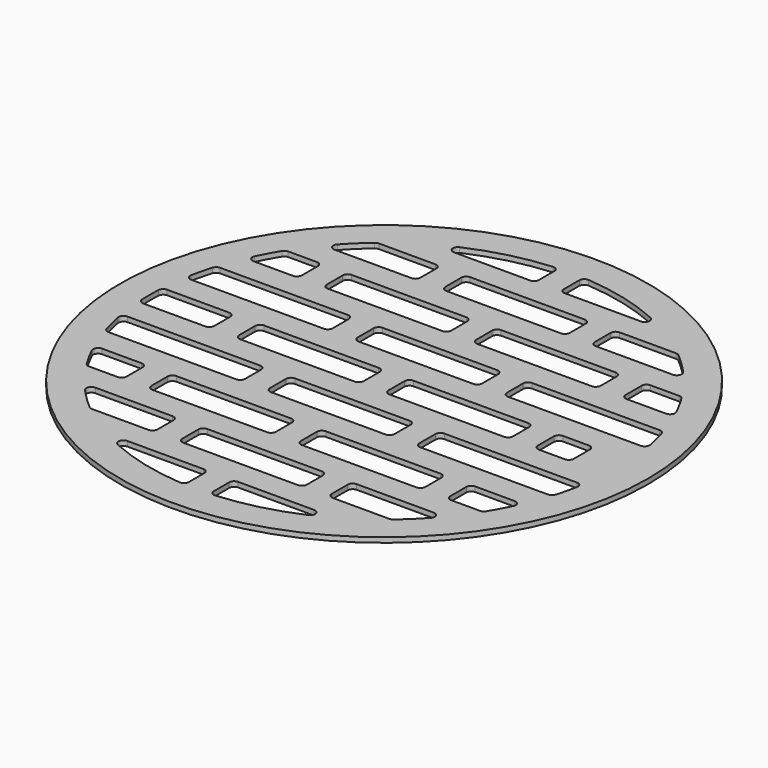
from build123d import *

# Parameters (mm, degrees)
F0_R     = 53
F0_W     = 25
F0_H     = 6
F0_W_2   = 7.2020787991
F1_DEPTH = 1
F2_R     = 1


with BuildPart() as f1:
    # F0 (on Top) → F1 (new body)
    with BuildSketch(Plane.XY):
        Circle(F0_R)
        with BuildLine():
            Line((-17.5, -30), (-17.5, -36))
            Line((-17.5, -36), (-30.2158898595, -36))
            ThreePointArc((-30.2158898595, -36), (-33.3332721818, -33.1344679398), (-36.1801050303, -30))
            Line((-36.1801050303, -30), (-17.5, -30))
        make_face(mode=Mode.SUBTRACT)
        with BuildLine():
            Line((-2.5, -41), (-2.5, -46.9334635415))
            ThreePointArc((-2.5, -46.9334635415), (-13.0800156969, -45.1432518697), (-22.9782505862, -41))
            Line((-22.9782505862, -41), (-2.5, -41))
        make_face(mode=Mode.SUBTRACT)
        with BuildLine():
            Line((-32.5, -25), (-39.7994974843, -25))
            ThreePointArc((-39.7994974843, -25), (-41.5025032039, -22.0577022332), (-42.9883705204, -19))
            Line((-42.9883705204, -19), (-32.5, -19))
            Line((-32.5, -19), (-32.5, -25))
        make_face(mode=Mode.SUBTRACT)
        with BuildLine():
            Line((-17.5, -14), (-44.8664685483, -14))
            ThreePointArc((-44.8664685483, -14), (-45.6889052007, -11.0237898005), (-46.3141447076, -8))
            Line((-46.3141447076, -8), (-17.5, -8))
            Line((-17.5, -8), (-17.5, -14))
        make_face(mode=Mode.SUBTRACT)
        with Locations((-15, -22)):
            Rectangle(F0_W, F0_H, mode=Mode.SUBTRACT)
        with BuildLine():
            ThreePointArc((22.9782505862, -41), (13.0800156969, -45.1432518697), (2.5, -46.9334635415))
            Line((2.5, -46.9334635415), (2.5, -41))
            Line((2.5, -41), (22.9782505862, -41))
        make_face(mode=Mode.SUBTRACT)
        with Locations((0, -33)):
            Rectangle(F0_W, F0_H, mode=Mode.SUBTRACT)
        with BuildLine():
            Line((30.2158898595, -36), (17.5, -36))
            Line((17.5, -36), (17.5, -30))
            Line((17.5, -30), (36.1801050303, -30))
            ThreePointArc((36.1801050303, -30), (33.3332721818, -33.1344679398), (30.2158898595, -36))
        make_face(mode=Mode.SUBTRACT)
        with Locations((15, -22)):
            Rectangle(F0_W, F0_H, mode=Mode.SUBTRACT)
        with Locations((0, -11)):
            Rectangle(F0_W, F0_H, mode=Mode.SUBTRACT)
        with BuildLine():
            Line((32.5, -19), (42.9883705204, -19))
            ThreePointArc((42.9883705204, -19), (41.5025032039, -22.0577022332), (39.7994974843, -25))
            Line((39.7994974843, -25), (32.5, -25))
            Line((32.5, -25), (32.5, -19))
        make_face(mode=Mode.SUBTRACT)
        with BuildLine():
            Line((17.5, -8), (46.3141447076, -8))
            ThreePointArc((46.3141447076, -8), (45.6889052007, -11.0237898005), (44.8664685483, -14))
            Line((44.8664685483, -14), (17.5, -14))
            Line((17.5, -14), (17.5, -8))
        make_face(mode=Mode.SUBTRACT)
        with BuildLine():
            Line((-32.5, -3), (-46.9041575982, -3))
            ThreePointArc((-46.9041575982, -3), (-47, 0), (-46.9041575982, 3))
            Line((-46.9041575982, 3), (-32.5, 3))
            Line((-32.5, 3), (-32.5, -3))
        make_face(mode=Mode.SUBTRACT)
        with BuildLine():
            Line((-17.5, 8), (-46.3141447076, 8))
            ThreePointArc((-46.3141447076, 8), (-45.6889052007, 11.0237898005), (-44.8664685483, 14))
            Line((-44.8664685483, 14), (-17.5, 14))
            Line((-17.5, 14), (-17.5, 8))
        make_face(mode=Mode.SUBTRACT)
        with BuildLine():
            Line((-32.5, 19), (-42.9883705204, 19))
            ThreePointArc((-42.9883705204, 19), (-41.5025032039, 22.0577022332), (-39.7994974843, 25))
            Line((-39.7994974843, 25), (-32.5, 25))
            Line((-32.5, 25), (-32.5, 19))
        make_face(mode=Mode.SUBTRACT)
        with Locations((-15, 0)):
            Rectangle(F0_W, F0_H, mode=Mode.SUBTRACT)
        with Locations((-15, 22)):
            Rectangle(F0_W, F0_H, mode=Mode.SUBTRACT)
        with BuildLine():
            Line((-17.5, 30), (-36.1801050303, 30))
            ThreePointArc((-36.1801050303, 30), (-33.3332721818, 33.1344679398), (-30.2158898595, 36))
            Line((-30.2158898595, 36), (-17.5, 36))
            Line((-17.5, 36), (-17.5, 30))
        make_face(mode=Mode.SUBTRACT)
        with BuildLine():
            ThreePointArc((-22.9782505862, 41), (-13.0800156969, 45.1432518697), (-2.5, 46.9334635415))
            Line((-2.5, 46.9334635415), (-2.5, 41))
            Line((-2.5, 41), (-22.9782505862, 41))
        make_face(mode=Mode.SUBTRACT)
        with Locations((0, 11)):
            Rectangle(F0_W, F0_H, mode=Mode.SUBTRACT)
        with Locations((15, 0)):
            Rectangle(F0_W, F0_H, mode=Mode.SUBTRACT)
        with Locations((15, 22)):
            Rectangle(F0_W, F0_H, mode=Mode.SUBTRACT)
        with Locations((36.1010393996, 0)):
            Rectangle(F0_W_2, F0_H, mode=Mode.SUBTRACT)
        with BuildLine():
            ThreePointArc((44.8664685483, 14), (45.6889052007, 11.0237898005), (46.3141447076, 8))
            Line((46.3141447076, 8), (17.5, 8))
            Line((17.5, 8), (17.5, 14))
            Line((17.5, 14), (44.8664685483, 14))
        make_face(mode=Mode.SUBTRACT)
        with BuildLine():
            ThreePointArc((39.7994974843, 25), (41.5025032039, 22.0577022332), (42.9883705204, 19))
            Line((42.9883705204, 19), (32.5, 19))
            Line((32.5, 19), (32.5, 25))
            Line((32.5, 25), (39.7994974843, 25))
        make_face(mode=Mode.SUBTRACT)
        with Locations((0, 33)):
            Rectangle(F0_W, F0_H, mode=Mode.SUBTRACT)
        with BuildLine():
            ThreePointArc((2.5, 46.9334635415), (13.0800156969, 45.1432518697), (22.9782505862, 41))
            Line((22.9782505862, 41), (2.5, 41))
            Line((2.5, 41), (2.5, 46.9334635415))
        make_face(mode=Mode.SUBTRACT)
        with BuildLine():
            ThreePointArc((30.2158898595, 36), (33.3332721818, 33.1344679398), (36.1801050303, 30))
            Line((36.1801050303, 30), (17.5, 30))
            Line((17.5, 30), (17.5, 36))
            Line((17.5, 36), (30.2158898595, 36))
        make_face(mode=Mode.SUBTRACT)
    extrude(amount=F1_DEPTH)

    # F2
    f2_edges = [f1.edges().sort_by_distance(p)[0] for p in [
        (22.978251, 41, 0.5),
        (-22.978251, 41, 0.5),
        (36.180105, 30, 0.5),
        (42.988371, 19, 0.5),
        (46.314145, 8, 0.5),
        (46.314145, -8, 0.5),
        (44.866469, -14, 0.5),
        (39.799497, -25, 0.5),
        (30.21589, -36, 0.5),
        (22.978251, -41, 0.5),
        (36.180105, -30, 0.5),
        (42.988371, -19, 0.5),
        (44.866469, 14, 0.5),
        (39.799497, 25, 0.5),
        (30.21589, 36, 0.5),
        (-2.5, 46.933464, 0.5),
        (-2.5, 41, 0.5),
        (2.5, 46.933464, 0.5),
        (2.5, 41, 0.5),
        (-36.180105, 30, 0.5),
        (-30.21589, 36, 0.5),
        (-17.5, 36, 0.5),
        (-17.5, 30, 0.5),
        (-2.5, 19, 0.5),
        (-32.5, 19, 0.5),
        (-32.5, 25, 0.5),
        (-39.799497, 25, 0.5),
        (-42.988371, 19, 0.5),
        (-27.5, 19, 0.5),
        (-27.5, 25, 0.5),
        (-2.5, 25, 0.5),
        (12.5, 36, 0.5),
        (-12.5, 36, 0.5),
        (-12.5, 30, 0.5),
        (12.5, 30, 0.5),
        (17.5, 30, 0.5),
        (17.5, 36, 0.5),
        (32.5, 25, 0.5),
        (32.5, 19, 0.5),
        (27.5, 19, 0.5),
        (27.5, 25, 0.5),
        (2.5, 25, 0.5),
        (2.5, 19, 0.5),
        (17.5, 14, 0.5),
        (17.5, 8, 0.5),
        (-12.5, 8, 0.5),
        (-46.314145, 8, 0.5),
        (-12.5, 14, 0.5),
        (-44.866469, 14, 0.5),
        (-17.5, 14, 0.5),
        (-17.5, 8, 0.5),
        (12.5, 8, 0.5),
        (12.5, 14, 0.5),
        (27.5, 3, 0.5),
        (27.5, -3, 0.5),
        (-2.5, -3, 0.5),
        (-2.5, 3, 0.5),
        (-32.5, 3, 0.5),
        (-32.5, -3, 0.5),
        (-46.904158, 3, 0.5),
        (-44.866469, -14, 0.5),
        (-46.904158, -3, 0.5),
        (-27.5, -3, 0.5),
        (2.5, -3, 0.5),
        (2.5, 3, 0.5),
        (-17.5, -8, 0.5),
        (-17.5, -14, 0.5),
        (-46.314145, -8, 0.5),
        (-12.5, -8, 0.5),
        (-12.5, -14, 0.5),
        (12.5, -14, 0.5),
        (12.5, -8, 0.5),
        (17.5, -8, 0.5),
        (17.5, -14, 0.5),
        (32.5, -19, 0.5),
        (32.5, -25, 0.5),
        (17.5, -36, 0.5),
        (17.5, -30, 0.5),
        (2.5, -19, 0.5),
        (27.5, -19, 0.5),
        (27.5, -25, 0.5),
        (2.5, -25, 0.5),
        (-12.5, -36, 0.5),
        (-30.21589, -36, 0.5),
        (-36.180105, -30, 0.5),
        (-17.5, -30, 0.5),
        (-17.5, -36, 0.5),
        (-2.5, -46.933464, 0.5),
        (-22.978251, -41, 0.5),
        (-2.5, -41, 0.5),
        (2.5, -41, 0.5),
        (2.5, -46.933464, 0.5),
        (-12.5, -30, 0.5),
        (12.5, -36, 0.5),
        (12.5, -30, 0.5),
        (-2.5, -19, 0.5),
        (-32.5, -19, 0.5),
        (-42.988371, -19, 0.5),
        (-27.5, -19, 0.5),
        (-39.799497, -25, 0.5),
        (-27.5, -25, 0.5),
        (-32.5, -25, 0.5),
        (-2.5, -25, 0.5),
        (-27.5, 3, 0.5),
        (32.5, -3, 0.5),
        (32.5, 3, 0.5),
        (39.702079, 3, 0.5),
        (39.702079, -3, 0.5),
    ]]
    fillet(f2_edges, radius=F2_R)


solid = f1.part
